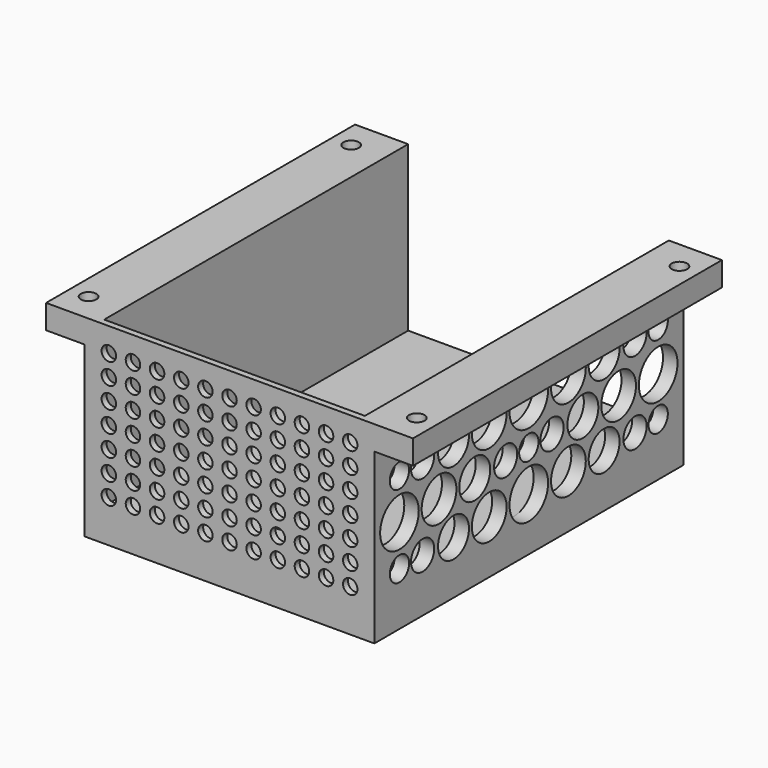
from build123d import *

# Parameters (mm, degrees)
F0_W     = 54
F0_H     = 1.3
F1_DEPTH = 40
F0_H_2   = 78.7
F0_R     = 1.75
F2_DEPTH = 6
F3_START = 35
F0_W_2   = 8
F0_H_3   = 80
F0_R_2   = 1.6
F3_DEPTH = 5
F4_R     = 2.5
F4_R_2   = 3
F4_R_3   = 4
F4_R_4   = 4.5
F4_R_5   = 5
F5_DEPTH = 5
F6_R     = 1.5
F7_DEPTH = 2


# Not quite as in the source:
# - a feature names something its author has since deleted; it is built from what else it names


with BuildPart() as f1:
    # F0 (on Top) → F1 (new body)
    with BuildSketch(Plane.XY):
        Polygon((-23.4806801195, 28.625481434), (-26.4806801195, 28.625481434), (-26.4806801195, -51.374518566), (-23.4806801195, -51.374518566), (-23.4806801195, -50.074518566), align=None)
        Polygon((33.5193198805, 28.625481434), (30.5193198805, 28.625481434), (30.5193198805, -50.074518566), (30.5193198805, -51.374518566), (33.5193198805, -51.374518566), align=None)
        with Locations((3.5193198805, -50.724518566)):
            Rectangle(F0_W, F0_H)
    extrude(amount=F1_DEPTH)

    # F0 (on Top) → F2 (join)
    with BuildSketch(Plane.XY):
        with Locations((3.5193198805, -10.724518566)):
            Rectangle(F0_W, F0_H_2)
        with Locations((3.5193198805, -37.074518566)):
            Circle(F0_R, mode=Mode.SUBTRACT)
        with Locations((3.5193198805, 17.425481434)):
            Circle(F0_R, mode=Mode.SUBTRACT)
    extrude(amount=F2_DEPTH)

    # F0 (on Top) → F3 (join)
    with BuildSketch(Plane.XY.offset(F3_START)):
        with Locations((-30.4806801195, -11.374518566)):
            Rectangle(F0_W_2, F0_H_3)
        with Locations((-30.4806801195, -45.374518566)):
            Circle(F0_R_2, mode=Mode.SUBTRACT)
        with Locations((-30.4806801195, 22.625481434)):
            Circle(F0_R_2, mode=Mode.SUBTRACT)
        with Locations((37.5193198805, -11.374518566)):
            Rectangle(F0_W_2, F0_H_3)
        with Locations((37.5193198805, -45.374518566)):
            Circle(F0_R_2, mode=Mode.SUBTRACT)
        with Locations((37.5193198805, 22.625481434)):
            Circle(F0_R_2, mode=Mode.SUBTRACT)
    extrude(amount=F3_DEPTH)

    # F4 (on face) → F5 (cut)
    with BuildSketch(Plane.YZ.offset(33.5193198805)):
        with Locations((-44.874518566, 28)):
            Circle(F4_R)
        with Locations((-38.874518566, 28)):
            Circle(F4_R_2)
        with Locations((-30.874518566, 28)):
            Circle(F4_R_3)
        with Locations((-21.624518566, 28)):
            Circle(F4_R_4)
        with Locations((-11.374518566, 28)):
            Circle(F4_R_5)
        with Locations((-11.374518566, 19.5)):
            Circle(F4_R)
        with Locations((-17.374518566, 19.5)):
            Circle(F4_R_2)
        with Locations((-25.374518566, 19.5)):
            Circle(F4_R_3)
        with Locations((-34.624518566, 19.5)):
            Circle(F4_R_4)
        with Locations((-44.874518566, 19.5)):
            Circle(F4_R_5)
        with Locations((-5.374518566, 19.5)):
            Circle(F4_R_2)
        with Locations((-1.124518566, 28)):
            Circle(F4_R_4)
        with Locations((2.625481434, 19.5)):
            Circle(F4_R_3)
        with Locations((11.875481434, 19.5)):
            Circle(F4_R_4)
        with Locations((8.125481434, 28)):
            Circle(F4_R_3)
        with Locations((16.125481434, 28)):
            Circle(F4_R_2)
        with Locations((22.125481434, 28)):
            Circle(F4_R)
        with Locations((22.125481434, 19.25)):
            Circle(F4_R_5)
        with Locations((-44.874518566, 11)):
            Circle(F4_R)
        with Locations((-38.874518566, 11)):
            Circle(F4_R_2)
        with Locations((-30.874518566, 11)):
            Circle(F4_R_3)
        with Locations((-21.624518566, 11)):
            Circle(F4_R_4)
        with Locations((-11.374518566, 11)):
            Circle(F4_R_5)
        with Locations((-1.124518566, 11)):
            Circle(F4_R_4)
        with Locations((8.125481434, 11)):
            Circle(F4_R_3)
        with Locations((16.125481434, 11)):
            Circle(F4_R_2)
        with Locations((22.125481434, 11)):
            Circle(F4_R)
    extrude(amount=-F5_DEPTH, mode=Mode.SUBTRACT)

    # F6 (on face) → F7 (cut)
    with BuildSketch(Plane.XZ.offset(51.374518566)):
        with Locations((-21.4806801195, 35)):
            Circle(F6_R)
        with Locations((-16.4806801195, 35)):
            Circle(F6_R)
        with Locations((-11.4806801195, 35)):
            Circle(F6_R)
        with Locations((-6.4806801195, 35)):
            Circle(F6_R)
        with Locations((-1.4806801195, 35)):
            Circle(F6_R)
        with Locations((3.5193198805, 35)):
            Circle(F6_R)
        with Locations((8.5193198805, 35)):
            Circle(F6_R)
        with Locations((13.5193198805, 35)):
            Circle(F6_R)
        with Locations((18.5193198805, 35)):
            Circle(F6_R)
        with Locations((23.5193198805, 35)):
            Circle(F6_R)
        with Locations((28.5193198805, 35)):
            Circle(F6_R)
        with Locations((-21.4806801195, 26.25)):
            Circle(F6_R)
        with Locations((-16.4806801195, 26.25)):
            Circle(F6_R)
        with Locations((-11.4806801195, 26.25)):
            Circle(F6_R)
        with Locations((-6.4806801195, 26.25)):
            Circle(F6_R)
        with Locations((-1.4806801195, 26.25)):
            Circle(F6_R)
        with Locations((3.5193198805, 26.25)):
            Circle(F6_R)
        with Locations((8.5193198805, 26.25)):
            Circle(F6_R)
        with Locations((13.5193198805, 26.25)):
            Circle(F6_R)
        with Locations((18.5193198805, 26.25)):
            Circle(F6_R)
        with Locations((23.5193198805, 26.25)):
            Circle(F6_R)
        with Locations((28.5193198805, 26.25)):
            Circle(F6_R)
        with Locations((-21.4806801195, 17.5)):
            Circle(F6_R)
        with Locations((-16.4806801195, 17.5)):
            Circle(F6_R)
        with Locations((-11.4806801195, 17.5)):
            Circle(F6_R)
        with Locations((-6.4806801195, 17.5)):
            Circle(F6_R)
        with Locations((-1.4806801195, 17.5)):
            Circle(F6_R)
        with Locations((3.5193198805, 17.5)):
            Circle(F6_R)
        with Locations((8.5193198805, 17.5)):
            Circle(F6_R)
        with Locations((13.5193198805, 17.5)):
            Circle(F6_R)
        with Locations((18.5193198805, 17.5)):
            Circle(F6_R)
        with Locations((23.5193198805, 17.5)):
            Circle(F6_R)
        with Locations((28.5193198805, 17.5)):
            Circle(F6_R)
        with Locations((28.5193198805, 8.75)):
            Circle(F6_R)
        with Locations((23.5193198805, 8.75)):
            Circle(F6_R)
        with Locations((18.5193198805, 8.75)):
            Circle(F6_R)
        with Locations((13.5193198805, 8.75)):
            Circle(F6_R)
        with Locations((8.5193198805, 8.75)):
            Circle(F6_R)
        with Locations((3.5193198805, 8.75)):
            Circle(F6_R)
        with Locations((-1.4806801195, 8.75)):
            Circle(F6_R)
        with Locations((-6.4806801195, 8.75)):
            Circle(F6_R)
        with Locations((-21.4806801195, 8.75)):
            Circle(F6_R)
        with Locations((-16.4806801195, 8.75)):
            Circle(F6_R)
        with Locations((-11.4806801195, 8.75)):
            Circle(F6_R)
        with Locations((8.5193198805, 30.625)):
            Circle(F6_R)
        with Locations((-21.4806801195, 30.625)):
            Circle(F6_R)
        with Locations((28.5193198805, 30.625)):
            Circle(F6_R)
        with Locations((-16.4806801195, 30.625)):
            Circle(F6_R)
        with Locations((23.5193198805, 30.625)):
            Circle(F6_R)
        with Locations((-6.4806801195, 30.625)):
            Circle(F6_R)
        with Locations((13.5193198805, 30.625)):
            Circle(F6_R)
        with Locations((-11.4806801195, 30.625)):
            Circle(F6_R)
        with Locations((18.5193198805, 30.625)):
            Circle(F6_R)
        with Locations((3.5193198805, 30.625)):
            Circle(F6_R)
        with Locations((-1.4806801195, 30.625)):
            Circle(F6_R)
        with Locations((8.5193198805, 21.875)):
            Circle(F6_R)
        with Locations((-11.4806801195, 21.875)):
            Circle(F6_R)
        with Locations((-6.4806801195, 21.875)):
            Circle(F6_R)
        with Locations((-16.4806801195, 21.875)):
            Circle(F6_R)
        with Locations((13.5193198805, 21.875)):
            Circle(F6_R)
        with Locations((28.5193198805, 21.875)):
            Circle(F6_R)
        with Locations((-21.4806801195, 21.875)):
            Circle(F6_R)
        with Locations((23.5193198805, 21.875)):
            Circle(F6_R)
        with Locations((18.5193198805, 21.875)):
            Circle(F6_R)
        with Locations((-1.4806801195, 21.875)):
            Circle(F6_R)
        with Locations((3.5193198805, 21.875)):
            Circle(F6_R)
        with Locations((3.5193198805, 13.125)):
            Circle(F6_R)
        with Locations((-1.4806801195, 13.125)):
            Circle(F6_R)
        with Locations((18.5193198805, 13.125)):
            Circle(F6_R)
        with Locations((28.5193198805, 13.125)):
            Circle(F6_R)
        with Locations((-6.4806801195, 13.125)):
            Circle(F6_R)
        with Locations((23.5193198805, 13.125)):
            Circle(F6_R)
        with Locations((-21.4806801195, 13.125)):
            Circle(F6_R)
        with Locations((13.5193198805, 13.125)):
            Circle(F6_R)
        with Locations((-16.4806801195, 13.125)):
            Circle(F6_R)
        with Locations((8.5193198805, 13.125)):
            Circle(F6_R)
        with Locations((-11.4806801195, 13.125)):
            Circle(F6_R)
    extrude(amount=-F7_DEPTH, mode=Mode.SUBTRACT)


solid = f1.part
